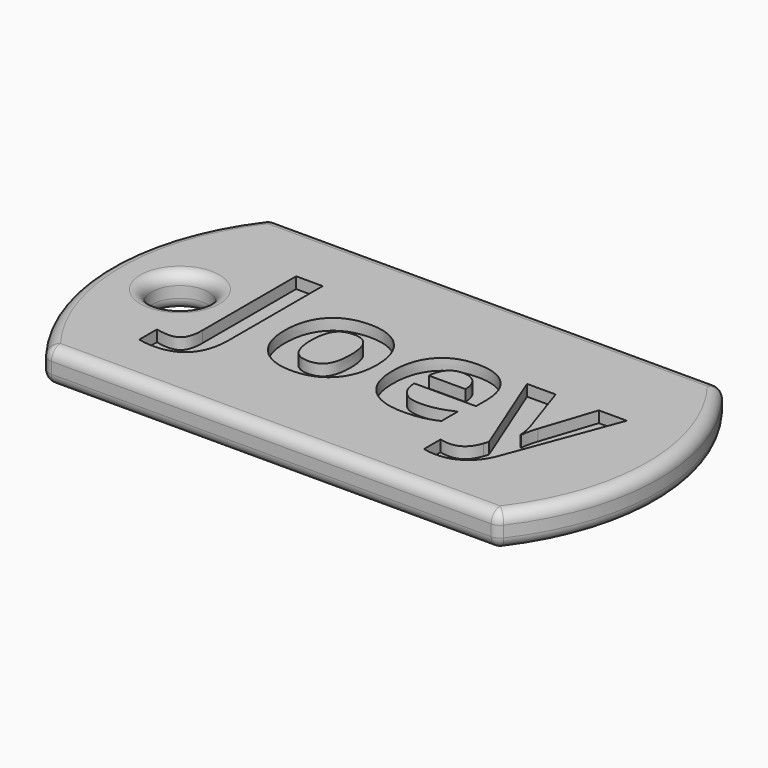
from build123d import *

# Parameters (mm, degrees)
F0_R         = 2.5
F1_DEPTH     = 3
F2_TEXT_SIZE = 15.5620397388
F3_DEPTH     = 1
F4_TEXT_SIZE = 11.5356885364
F5_DEPTH     = 1
F6_R         = 1


# Not quite as in the source:
# - Text() gives the source's letters only with a copy of the font that has no kerning and outlines rounded to 1/6400 em; it was checked with that copy


with BuildPart() as f1:
    # F0 (on Top) → F1 (new body)
    with BuildSketch(Plane.XY):
        with BuildLine():
            Line((20, 12.5), (-20, 12.5))
            ThreePointArc((-20, 12.5), (-24.387505004, 0), (-20, -12.5))
            Line((-20, -12.5), (20, -12.5))
            ThreePointArc((20, -12.5), (24.387505004, 0), (20, 12.5))
        make_face()
        with Locations((-18.112494996, 0)):
            Circle(F0_R, mode=Mode.SUBTRACT)
    extrude(amount=F1_DEPTH)

    # F2 (on face) → F3 (cut)
    with BuildSketch(Plane.XY.offset(3)):
        with Locations((-14.4549424787, -4.5377247157)):
            Text('Joey', F2_TEXT_SIZE, font='Open Sans', font_style=FontStyle.BOLD, text_align=(TextAlign.LEFT, TextAlign.BOTTOM))
    extrude(amount=-F3_DEPTH, mode=Mode.SUBTRACT)

    # F4 (on face) → F5 (cut)
    with BuildSketch(Plane(origin=(0, 0, 0), x_dir=(1, 0, 0), z_dir=(0, 0, -1))):
        with Locations((-13.4398699892, -3.8352218119)):
            Text('Braun', F4_TEXT_SIZE, font='Open Sans', font_style=FontStyle.BOLD, text_align=(TextAlign.LEFT, TextAlign.BOTTOM))
    extrude(amount=-F5_DEPTH, mode=Mode.SUBTRACT)

    # F6
    f6_edges = [f1.edges().sort_by_distance(p)[0] for p in [
        (20, -12.5, 1.5),
        (20, 12.5, 1.5),
        (24.387505, 0, 0),
        (24.387505, 0, 3),
        (-20, -12.5, 1.5),
        (0, -12.5, 0),
        (0, -12.5, 3),
        (-15.612495, 0, 1.5),
        (-20.612495, 0, 0),
        (-20.612495, 0, 3),
        (-20, 12.5, 1.5),
        (-24.387505, 0, 0),
        (-24.387505, 0, 3),
        (0, 12.5, 0),
        (0, 12.5, 3),
    ]]
    fillet(f6_edges, radius=F6_R)


solid = f1.part
